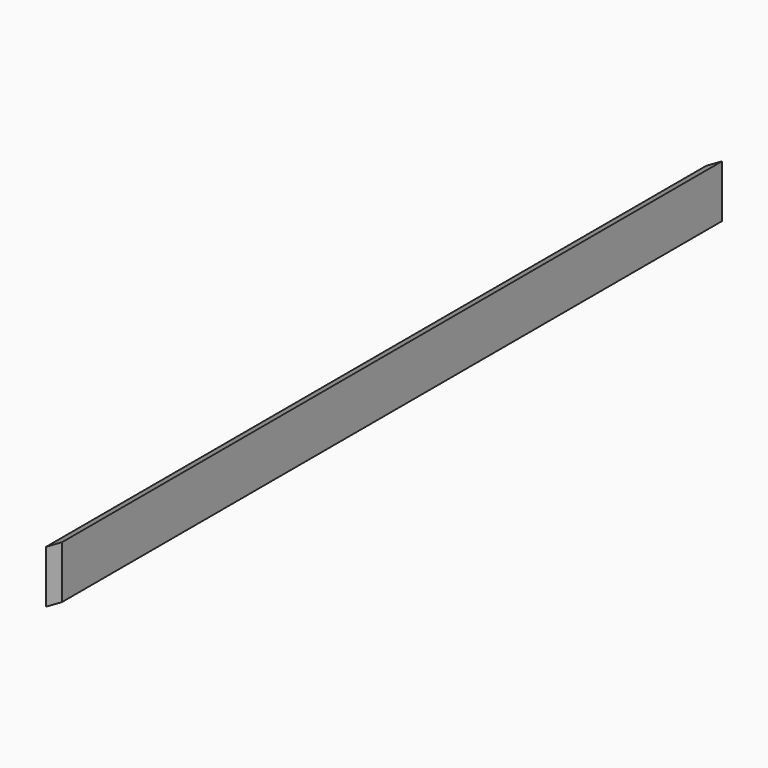
from build123d import *

# Parameters (mm, degrees)
F1_DEPTH = 90


# Not quite as in the source:
# - a feature names something its author has since deleted; it is built from what else it names


with BuildPart() as f1:
    # F0 (on Front) → F1 (new body)
    with BuildSketch(Plane.XZ):
        Polygon((0, 5.75), (0, 0), (1.7320508076, 1), (1.7320508076, 6.75), align=None)
    extrude(amount=F1_DEPTH)


solid = f1.part
